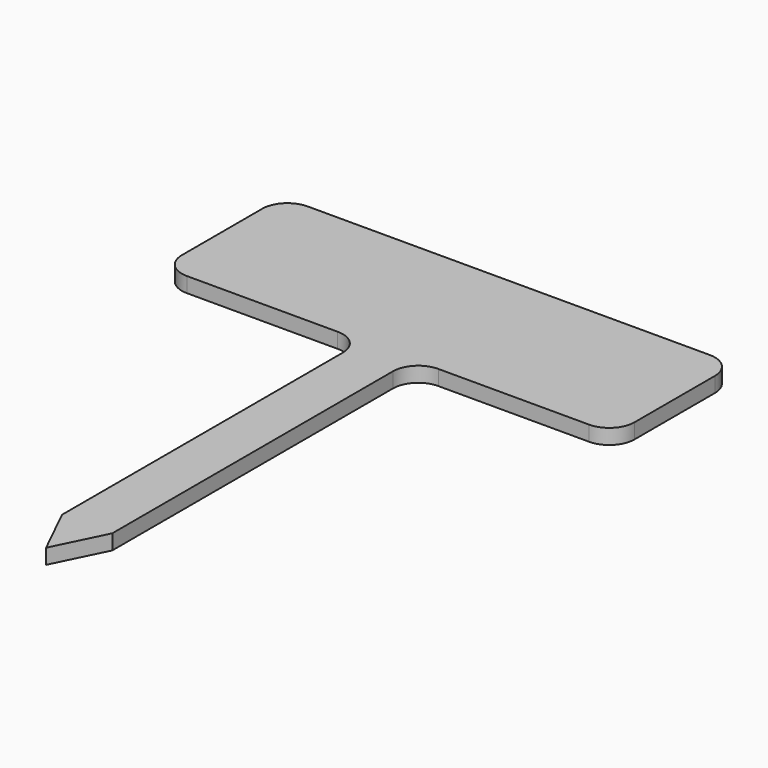
from build123d import *

# Parameters (mm, degrees)
F0_W     = 10
F0_H     = 85
F1_DEPTH = 3
F2_R     = 5
F4_DEPTH = 25


# Not quite as in the source:
# - a feature names something its author has since deleted; it is built from what else it names


with BuildPart() as f1:
    # F0 (on Top) → F1 (new body)
    with BuildSketch(Plane.XY):
        Polygon((45, 30), (-45, 30), (-45, 0), (-5, 0), (5, 0), (45, 0), align=None)
        with Locations((0, -42.5)):
            Rectangle(F0_W, F0_H)
    extrude(amount=F1_DEPTH)

    # F2
    f2_edges = [f1.edges().sort_by_distance(p)[0] for p in [
        (-45, 0, 1.5),
        (-45, 30, 1.5),
        (45, 0, 1.5),
        (45, 30, 1.5),
        (5, 0, 1.5),
        (-5, 0, 1.5),
    ]]
    fillet(f2_edges, radius=F2_R)

    # F3 (on face) → F4 (cut)
    with BuildSketch(Plane.XY.offset(3)):
        Polygon((-5, -85), (0, -85), (-5, -74.790418148), align=None)
        Polygon((5, -74.790418148), (0, -85), (5, -85), align=None)
    extrude(amount=-F4_DEPTH, mode=Mode.SUBTRACT)


solid = f1.part
